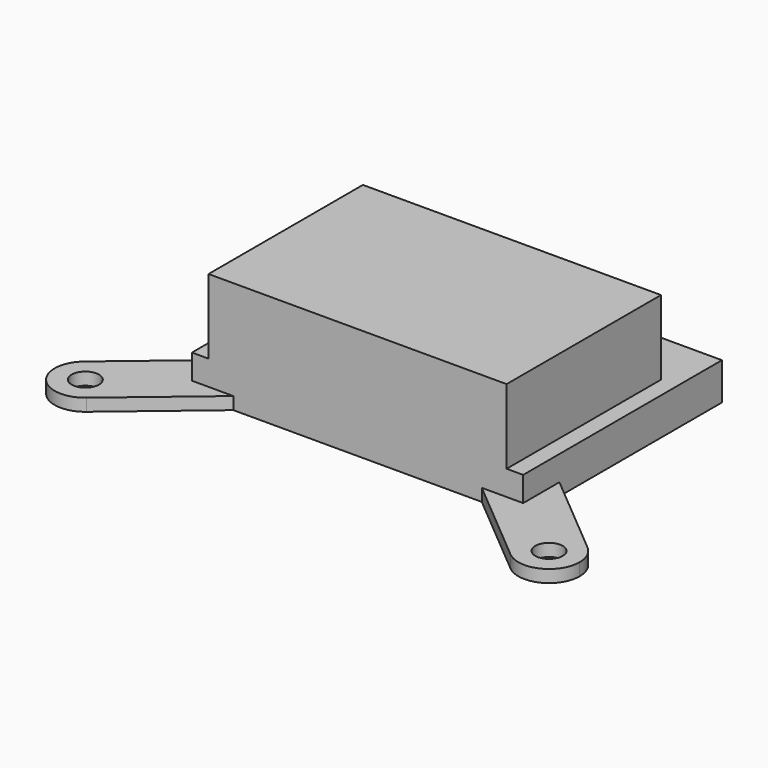
from build123d import *
from build123d import SkipClean  # not in build123d's __all__

# Parameters (mm, degrees)
F0_R     = 1.65
F1_DEPTH = 1.5
F3_DEPTH = 1.501
F4_DEPTH = 1.5
F5_W     = 40
F5_H     = 30
F6_DEPTH = 3
F7_W     = 36
F7_H     = 23.3
F8_DEPTH = 9


with BuildPart() as f1:
    # F0 (on Top) → F1 (new body)
    with BuildSketch(Plane.XY):
        with BuildLine():
            ThreePointArc((-0.73370891, 14), (-0.4891889552, 6.9935887205), (0, 0))
            Line((0, 0), (65, 0))
            ThreePointArc((65, 0), (65.4891889552, 6.9935887205), (65.73370891, 14))
            ThreePointArc((65.73370891, 14), (65.7334108185, 21.0021379582), (65.488741818, 28))
            Line((65.488741818, 28), (57.299411547, 50.5))
            ThreePointArc((57.299411547, 50.5), (32.5, 63.5), (7.700588453, 50.5))
            Line((7.700588453, 50.5), (-0.488741818, 28))
            ThreePointArc((-0.488741818, 28), (-0.7334108185, 21.0021379582), (-0.73370891, 14))
        make_face()
        with Locations((4.5, 12.5)):
            Circle(F0_R, mode=Mode.SUBTRACT)
        with Locations((60.5, 12.5)):
            Circle(F0_R, mode=Mode.SUBTRACT)
        with Locations((15, 54.5)):
            Circle(F0_R, mode=Mode.SUBTRACT)
    extrude(amount=F1_DEPTH)

    # F2 (on face) → F3 (cut, through all)
    with BuildSketch(Plane.XY.offset(1.5)):
        with BuildLine():
            ThreePointArc((15.3946260476, 58.178895253), (17.4713893755, 57.2535857631), (18.6149922575, 55.2885626028))
            Line((18.6149922575, 55.2885626028), (20.0740134556, 48.6))
            Line((20.0740134556, 48.6), (52.5, 48.6))
            Line((52.5, 48.6), (52.5, 24.064025175))
            Line((52.5, 24.064025175), (62.8817094627, 15.3315119698))
            ThreePointArc((62.8817094627, 15.3315119698), (63.8542752579, 14.0616777817), (64.2, 12.5))
            ThreePointArc((64.2, 12.5), (62.0616777817, 9.1457247421), (58.1182905373, 9.6684880302))
            Line((58.1182905373, 9.6684880302), (47.5, 18.6))
            Line((47.5, 18.6), (17.5, 18.6))
            Line((17.5, 18.6), (6.8817094627, 9.6684880302))
            ThreePointArc((6.8817094627, 9.6684880302), (1.6684880302, 10.1182905373), (2.1182905373, 15.3315119698))
            Line((2.1182905373, 15.3315119698), (12.5, 24.064025175))
            Line((12.5, 24.064025175), (12.5, 48.6))
            Line((12.5, 48.6), (11.3850077425, 53.7114373972))
            ThreePointArc((11.3850077425, 53.7114373972), (11.308192582, 54.2539146721), (11.3123280961, 54.8017878876))
            ThreePointArc((11.3123280961, 54.8017878876), (9.4060764304, 52.7351735725), (7.700588453, 50.5))
            Line((7.700588453, 50.5), (-0.488741818, 28))
            ThreePointArc((-0.488741818, 28), (-0.733560046, 13.9914611719), (0, 0))
            Line((0, 0), (65, 0))
            ThreePointArc((65, 0), (65.733560046, 13.9914611719), (65.488741818, 28))
            Line((65.488741818, 28), (57.299411547, 50.5))
            ThreePointArc((57.299411547, 50.5), (37.9351551683, 63.0061258111), (15.3946260476, 58.178895253))
        make_face()
    extrude(amount=-F3_DEPTH, mode=Mode.SUBTRACT)

    # F2 (on face) → F4 (join)
    with BuildSketch(Plane.XY.offset(1.5)):
        with BuildLine():
            ThreePointArc((11.3123280961, 54.8017878876), (13.2791635515, 56.5801728664), (15.3946260476, 58.178895253))
            ThreePointArc((15.3946260476, 58.178895253), (12.6415574435, 57.3509206772), (11.3123280961, 54.8017878876))
        make_face()
    with SkipClean():  # cleaning this boolean's faces spoils the solid; the shape is the same uncleaned
        extrude(amount=-F4_DEPTH)

    # F5 (on face) → F6 (join)
    with BuildSketch(Plane.XY.offset(1.5)):
        with Locations((32.5, 33.6)):
            Rectangle(F5_W, F5_H)
    extrude(amount=F6_DEPTH)

    # F7 (on face) → F8 (join)
    with BuildSketch(Plane.XY.offset(4.5)):
        with Locations((32.5, 30.25)):
            Rectangle(F7_W, F7_H)
    extrude(amount=F8_DEPTH)


solid = f1.part
